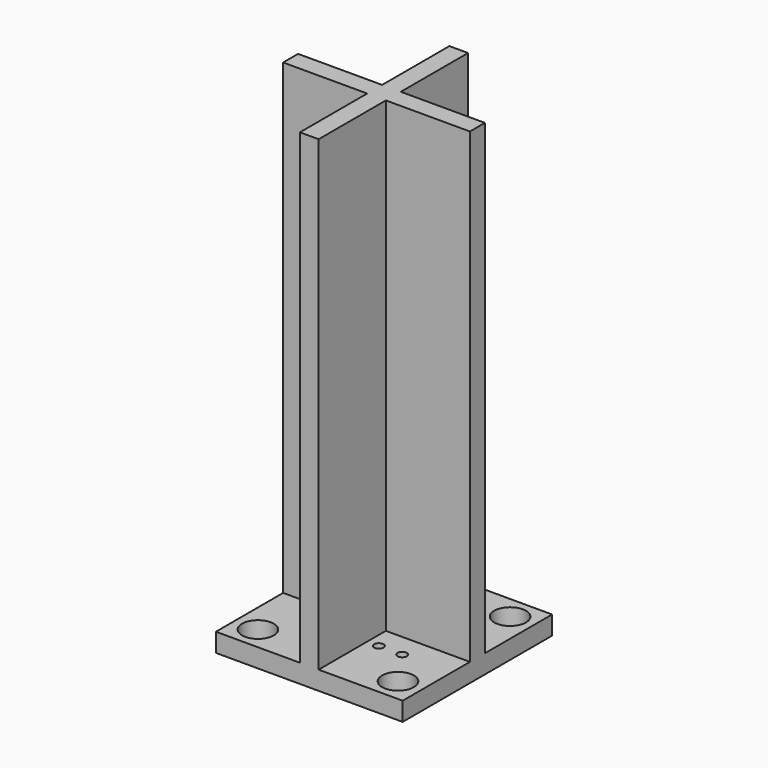
from build123d import *

# Parameters (mm, degrees)
F1_DEPTH = 1
F3_D     = 1
F4_W     = 2
F4_H     = 9
F4_H_2   = 2
F4_W_2   = 9
F5_DEPTH = 50
F6_D     = 3.4


# Not quite as in the source:
# - a feature names something its author has since deleted; it is built from what else it names


with BuildPart() as f1:
    # F0 (on Top) → F1 (new body, symmetric)
    with BuildSketch(Plane.XY):
        Polygon((10, 1), (10, 10), (1, 10), (-1, 10), (-10, 10), (-10, 1), (-10, -1), (-10, -10), (-1, -10), (1, -10), (10, -10), (10, -1), align=None)
    extrude(amount=F1_DEPTH, both=True)

    # F3 (through all)
    with Locations(Plane.XY.offset(1)):
        with Locations((-4.75, 3.5), (-2.25, 3.5), (-4.75, -3.5), (-2.25, -3.5), (2.25, 3.5), (4.75, 3.5), (4.75, -3.5), (2.25, -3.5)):
            Hole(F3_D / 2)

    # F4 (on face) → F5 (join)
    with BuildSketch(Plane.XY.offset(1)):
        with Locations((0, 5.5)):
            Rectangle(F4_W, F4_H)
        Rectangle(F4_W, F4_H_2)
        with Locations((-5.5, 0)):
            Rectangle(F4_W_2, F4_H_2)
        with Locations((5.5, 0)):
            Rectangle(F4_W_2, F4_H_2)
        with Locations((0, -5.5)):
            Rectangle(F4_W, F4_H)
    extrude(amount=F5_DEPTH)

    # F6 (through all)
    with Locations(Plane.XY.offset(1)):
        with Locations((-7.5, 7.5), (7.5, 7.5), (7.5, -7.5), (-7.5, -7.5)):
            Hole(F6_D / 2)


solid = f1.part
